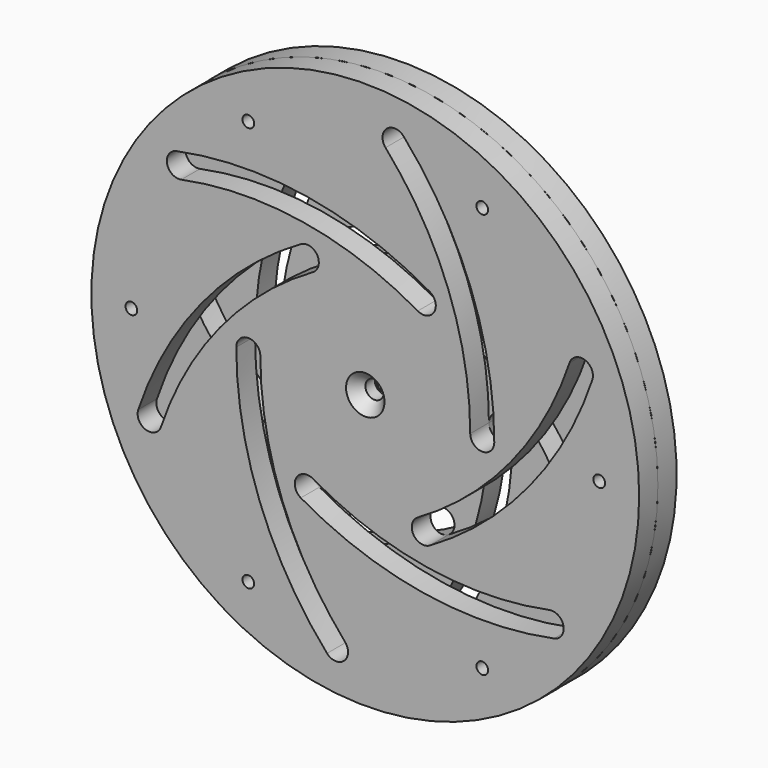
from build123d import *

# Parameters (mm, degrees)
F0_R              = 74.3458
F0_R_2            = 1.5875
F1_DEPTH          = 6.35
F2_DEPTH          = 6.35
F3_ANGLE          = 180
F5_D              = 4.9784
F5_CSINK_D        = 10.4394
F5_CSINK_ANGLE    = 82
F6_D              = 4.0386
F7_R              = 25.4
F8_DEPTH          = 6.35
F9_D              = 4.9784
F9_CSINK_D        = 10.4394
F9_CSINK_ANGLE    = 82
F11_D             = 4.9784
F11_CSINK_D       = 10.4394
F11_CSINK_ANGLE   = 82
F11_2_D           = 4.9784
F11_2_CSINK_D     = 10.4394
F11_2_CSINK_ANGLE = 82


# Not quite as in the source:
# - a feature names something its author has since deleted; it is built from what else it names


with BuildPart() as f1:
    # F0 (on Front) → F1 (new body)
    with BuildSketch(Plane.XZ):
        Circle(F0_R)
        with Locations((-31.75, -54.9926131403)):
            Circle(F0_R_2, mode=Mode.SUBTRACT)
        with BuildLine():
            ThreePointArc((-5.489575, -60.8430861687), (-5.778633074, -65.4498780947), (-10.385425, -65.1608200208))
            ThreePointArc((-10.385425, -65.1608200208), (-28.6513154087, -34.8299233656), (-35.0139, 0))
            ThreePointArc((-35.0139, 0), (-31.75, 3.2639), (-28.4861, 0))
            ThreePointArc((-28.4861, 0), (-22.5451176364, -32.5219975425), (-5.489575, -60.8430861687))
        make_face(mode=Mode.SUBTRACT)
        with Locations((31.75, -54.9926131403)):
            Circle(F0_R_2, mode=Mode.SUBTRACT)
        with BuildLine():
            ThreePointArc((49.9468707667, -35.1756544903), (53.7919405676, -37.7293820886), (51.2382129694, -41.5744518895))
            ThreePointArc((51.2382129694, -41.5744518895), (15.8379407421, -42.2277286786), (-17.50695, -30.3229268856))
            ThreePointArc((-17.50695, -30.3229268856), (-18.7016203154, -25.8643565702), (-14.24305, -24.6696862547))
            ThreePointArc((-14.24305, -24.6696862547), (16.8923172354, -35.7856433756), (49.9468707667, -35.1756544903))
        make_face(mode=Mode.SUBTRACT)
        with BuildLine():
            ThreePointArc((14.24305, -24.6696862547), (39.4374348718, -3.2636458332), (55.4364457667, 25.6674316784))
            ThreePointArc((55.4364457667, 25.6674316784), (59.5705736416, 27.7204960062), (61.6236379694, 23.5863681313))
            ThreePointArc((61.6236379694, 23.5863681313), (44.4892561508, -7.397805313), (17.50695, -30.3229268856))
            ThreePointArc((17.50695, -30.3229268856), (13.0483796846, -29.1282565702), (14.24305, -24.6696862547))
        make_face(mode=Mode.SUBTRACT)
        with Locations((-63.5, 0)):
            Circle(F0_R_2, mode=Mode.SUBTRACT)
        with BuildLine():
            ThreePointArc((-55.4364457667, -25.6674316784), (-59.5705736416, -27.7204960062), (-61.6236379694, -23.5863681313))
            ThreePointArc((-61.6236379694, -23.5863681313), (-44.4892561508, 7.397805313), (-17.50695, 30.3229268856))
            ThreePointArc((-17.50695, 30.3229268856), (-13.0483796846, 29.1282565702), (-14.24305, 24.6696862547))
            ThreePointArc((-14.24305, 24.6696862547), (-39.4374348718, 3.2636458332), (-55.4364457667, -25.6674316784))
        make_face(mode=Mode.SUBTRACT)
        with BuildLine():
            ThreePointArc((-49.9468707667, 35.1756544903), (-53.7919405676, 37.7293820886), (-51.2382129694, 41.5744518895))
            ThreePointArc((-51.2382129694, 41.5744518895), (-15.8379407421, 42.2277286786), (17.50695, 30.3229268856))
            ThreePointArc((17.50695, 30.3229268856), (18.7016203154, 25.8643565702), (14.24305, 24.6696862547))
            ThreePointArc((14.24305, 24.6696862547), (-16.8923172354, 35.7856433756), (-49.9468707667, 35.1756544903))
        make_face(mode=Mode.SUBTRACT)
        with Locations((-31.75, 54.9926131403)):
            Circle(F0_R_2, mode=Mode.SUBTRACT)
        with BuildLine():
            ThreePointArc((5.489575, 60.8430861687), (5.778633074, 65.4498780947), (10.385425, 65.1608200208))
            ThreePointArc((10.385425, 65.1608200208), (28.6513154087, 34.8299233656), (35.0139, 0))
            ThreePointArc((35.0139, 0), (31.75, -3.2639), (28.4861, 0))
            ThreePointArc((28.4861, 0), (22.5451176364, 32.5219975425), (5.489575, 60.8430861687))
        make_face(mode=Mode.SUBTRACT)
        with Locations((63.5, 0)):
            Circle(F0_R_2, mode=Mode.SUBTRACT)
        with Locations((31.75, 54.9926131403)):
            Circle(F0_R_2, mode=Mode.SUBTRACT)
    extrude(amount=F1_DEPTH)

    # F5 (through all)
    with Locations(Plane.XZ.offset(6.35)):
        with Locations((0, 0)):
            CounterSinkHole(F5_D / 2, F5_CSINK_D / 2, counter_sink_angle=F5_CSINK_ANGLE)


with BuildPart() as f2:
    # F0 (on Front) → F2 (new body, through all)
    with BuildSketch(Plane.XZ):
        Circle(F0_R)
        with Locations((-31.75, -54.9926131403)):
            Circle(F0_R_2, mode=Mode.SUBTRACT)
        with BuildLine():
            ThreePointArc((-5.489575, -60.8430861687), (-5.778633074, -65.4498780947), (-10.385425, -65.1608200208))
            ThreePointArc((-10.385425, -65.1608200208), (-28.6513154087, -34.8299233656), (-35.0139, 0))
            ThreePointArc((-35.0139, 0), (-31.75, 3.2639), (-28.4861, 0))
            ThreePointArc((-28.4861, 0), (-22.5451176364, -32.5219975425), (-5.489575, -60.8430861687))
        make_face(mode=Mode.SUBTRACT)
        with Locations((31.75, -54.9926131403)):
            Circle(F0_R_2, mode=Mode.SUBTRACT)
        with BuildLine():
            ThreePointArc((49.9468707667, -35.1756544903), (53.7919405676, -37.7293820886), (51.2382129694, -41.5744518895))
            ThreePointArc((51.2382129694, -41.5744518895), (15.8379407421, -42.2277286786), (-17.50695, -30.3229268856))
            ThreePointArc((-17.50695, -30.3229268856), (-18.7016203154, -25.8643565702), (-14.24305, -24.6696862547))
            ThreePointArc((-14.24305, -24.6696862547), (16.8923172354, -35.7856433756), (49.9468707667, -35.1756544903))
        make_face(mode=Mode.SUBTRACT)
        with BuildLine():
            ThreePointArc((14.24305, -24.6696862547), (39.4374348718, -3.2636458332), (55.4364457667, 25.6674316784))
            ThreePointArc((55.4364457667, 25.6674316784), (59.5705736416, 27.7204960062), (61.6236379694, 23.5863681313))
            ThreePointArc((61.6236379694, 23.5863681313), (44.4892561508, -7.397805313), (17.50695, -30.3229268856))
            ThreePointArc((17.50695, -30.3229268856), (13.0483796846, -29.1282565702), (14.24305, -24.6696862547))
        make_face(mode=Mode.SUBTRACT)
        with Locations((-63.5, 0)):
            Circle(F0_R_2, mode=Mode.SUBTRACT)
        with BuildLine():
            ThreePointArc((-55.4364457667, -25.6674316784), (-59.5705736416, -27.7204960062), (-61.6236379694, -23.5863681313))
            ThreePointArc((-61.6236379694, -23.5863681313), (-44.4892561508, 7.397805313), (-17.50695, 30.3229268856))
            ThreePointArc((-17.50695, 30.3229268856), (-13.0483796846, 29.1282565702), (-14.24305, 24.6696862547))
            ThreePointArc((-14.24305, 24.6696862547), (-39.4374348718, 3.2636458332), (-55.4364457667, -25.6674316784))
        make_face(mode=Mode.SUBTRACT)
        with BuildLine():
            ThreePointArc((-49.9468707667, 35.1756544903), (-53.7919405676, 37.7293820886), (-51.2382129694, 41.5744518895))
            ThreePointArc((-51.2382129694, 41.5744518895), (-15.8379407421, 42.2277286786), (17.50695, 30.3229268856))
            ThreePointArc((17.50695, 30.3229268856), (18.7016203154, 25.8643565702), (14.24305, 24.6696862547))
            ThreePointArc((14.24305, 24.6696862547), (-16.8923172354, 35.7856433756), (-49.9468707667, 35.1756544903))
        make_face(mode=Mode.SUBTRACT)
        with Locations((-31.75, 54.9926131403)):
            Circle(F0_R_2, mode=Mode.SUBTRACT)
        with BuildLine():
            ThreePointArc((5.489575, 60.8430861687), (5.778633074, 65.4498780947), (10.385425, 65.1608200208))
            ThreePointArc((10.385425, 65.1608200208), (28.6513154087, 34.8299233656), (35.0139, 0))
            ThreePointArc((35.0139, 0), (31.75, -3.2639), (28.4861, 0))
            ThreePointArc((28.4861, 0), (22.5451176364, 32.5219975425), (5.489575, 60.8430861687))
        make_face(mode=Mode.SUBTRACT)
        with Locations((63.5, 0)):
            Circle(F0_R_2, mode=Mode.SUBTRACT)
        with Locations((31.75, 54.9926131403)):
            Circle(F0_R_2, mode=Mode.SUBTRACT)
    extrude(amount=F2_DEPTH)


with BuildPart() as f2_1:
    # F3: moved
    add(f2.part.rotate(Axis((0, 0, 37.1729), (0, 0, 1)), F3_ANGLE))

    # F6 (through all)
    with Locations(Plane.XZ):
        with Locations((0, 0)):
            Hole(F6_D / 2)

    # F11 (through all)
    with Locations(Plane.XZ):
        with Locations((0, 19.05), (16.4977839421, -9.525), (-16.4977839421, -9.525)):
            CounterSinkHole(F11_D / 2, F11_CSINK_D / 2, counter_sink_angle=F11_CSINK_ANGLE)


with BuildPart() as f8:
    # F7 (on face) → F8 (new body)
    with BuildSketch(Plane(origin=(0, 6.35, 0), x_dir=(-1, 0, 0), z_dir=(0, 1, 0))):
        Circle(F7_R)
    extrude(amount=F8_DEPTH)

    # F9 (through all)
    with Locations(Plane(origin=(0, 6.35, 0), x_dir=(-1, 0, 0), z_dir=(0, -1, 0))):
        with Locations((0, 0)):
            CounterSinkHole(F9_D / 2, F9_CSINK_D / 2, counter_sink_angle=F9_CSINK_ANGLE)

    # F11#2 (through all)
    with Locations(Plane.XZ):
        with Locations((0, 19.05), (16.4977839421, -9.525), (-16.4977839421, -9.525)):
            CounterSinkHole(F11_2_D / 2, F11_2_CSINK_D / 2, counter_sink_angle=F11_2_CSINK_ANGLE)


solid = Compound([f1.part, f2_1.part, f8.part])
